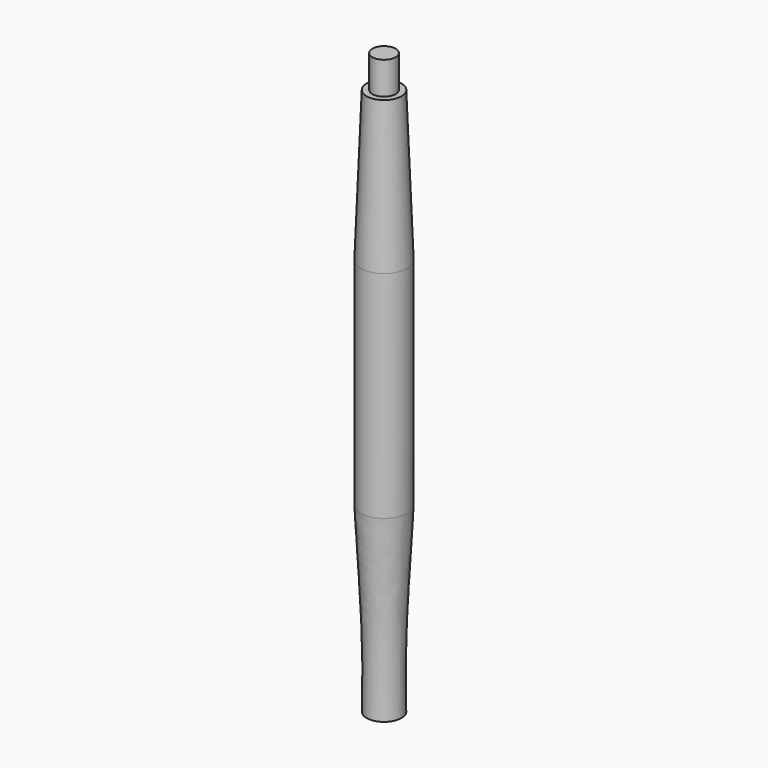
from build123d import *


# Not quite as in the source:
# - a feature names something its author has since deleted; it is built from what else it names


with BuildPart() as f1:
    # F0 (on Front) → F1 (revolve)
    with BuildSketch(Plane.XZ):
        with BuildLine():
            Line((0, 250), (0, 0))
            Line((0, 0), (0, -250))
            Line((0, -250), (15, -250))
            add(Edge.make_bspline(
                [(15, -250), (13.4045789018, -193.5875862837), (17.3846632242, -147.1532583237), (20, -92.9462272166)],
                knots=[0, 0, 0, 0, 157.1333432009, 157.1333432009, 157.1333432009, 157.1333432009], degree=3))
            Line((20, -92.9462272166), (20, 0))
            Line((20, 0), (20, 92.9462272166))
            add(Edge.make_bspline(
                [(15, 222), (16.6666666667, 181.3154090722), (18.3333333333, 133.6308181444), (20, 92.9462272166)],
                knots=[0, 0, 0, 0, 129.1505953127, 129.1505953127, 129.1505953127, 129.1505953127], degree=3))
            Line((15, 222), (10, 222))
            Line((10, 222), (10, 250))
            Line((10, 250), (0, 250))
        make_face()
    revolve(axis=Axis((0, 0, 125), (0, 0, 1)))


solid = f1.part
